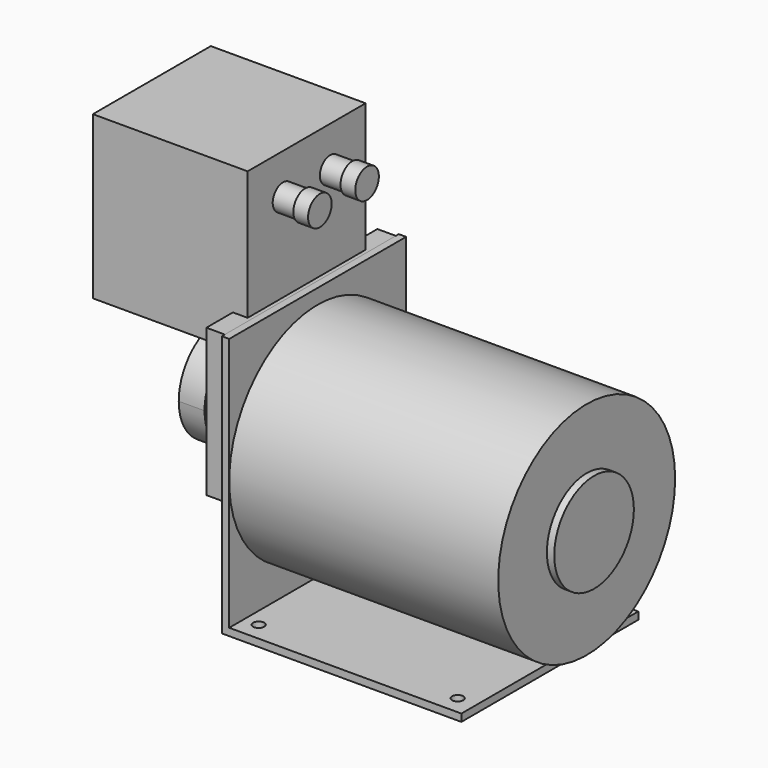
from build123d import *

# Parameters (mm, degrees)
F0_W      = 65
F0_H      = 60
F1_DEPTH  = 2
F2_W      = 2
F2_H      = 60
F3_DEPTH  = 69
F5_DEPTH  = 73
F6_R      = 13.5
F7_DEPTH  = 2
F8_W      = 58
F8_H      = 40
F9_DEPTH  = 5
F10_W     = 38
F10_H     = 27
F11_DEPTH = 5
F12_W     = 40
F12_H     = 44
F13_DEPTH = 38
F14_W     = 40
F14_H     = 35
F15_DEPTH = 4
F16_R     = 3.5
F17_DEPTH = 6
F18_R     = 4
F19_DEPTH = 4
F22_DEPTH = 3.5
F23_R     = 5
F24_DEPTH = 2
F25_R     = 12.5
F26_DEPTH = 12
F28_R     = 4
F29_DEPTH = 5
F30_R     = 1.5
F31_DEPTH = 25


with BuildPart() as f1:
    # F0 (on Top) → F1 (new body)
    with BuildSketch(Plane.XY):
        Rectangle(F0_W, F0_H)
    extrude(amount=F1_DEPTH)

    # F2 (on face) → F3 (join)
    with BuildSketch(Plane.XY.offset(2)):
        with Locations((-31.5, 0)):
            Rectangle(F2_W, F2_H)
    extrude(amount=F3_DEPTH)

    # F30 (on face) → F31 (cut)
    with BuildSketch(Plane(origin=(0, 0, 0), x_dir=(1, 0, 0), z_dir=(0, 0, -1))):
        with Locations((27.5, 25)):
            Circle(F30_R)
        with Locations((27.5, -25)):
            Circle(F30_R)
        with Locations((-26.5, 25)):
            Circle(F30_R)
        with Locations((-26.5, -25)):
            Circle(F30_R)
    extrude(amount=-F31_DEPTH, mode=Mode.SUBTRACT)


with BuildPart() as f5:
    # F4 (on face) → F5 (new body)
    with BuildSketch(Plane.YZ.offset(-30.5)):
        with BuildLine():
            ThreePointArc((-30, 37), (0, 7), (30, 37))
            ThreePointArc((30, 37), (0, 67), (-30, 37))
        make_face()
    extrude(amount=F5_DEPTH)

    # F6 (on face) → F7 (join)
    with BuildSketch(Plane.YZ.offset(42.5)):
        with Locations((0, 37)):
            Circle(F6_R)
    extrude(amount=F7_DEPTH)


with BuildPart() as f9:
    # F8 (on face) → F9 (new body)
    with BuildSketch(Plane(origin=(-32.5, 0, 0), x_dir=(0, -1, 0), z_dir=(-1, 0, 0))):
        with Locations((0, 51)):
            Rectangle(F8_W, F8_H)
    extrude(amount=F9_DEPTH)

    # F10 (on face) → F11 (cut, through all)
    with BuildSketch(Plane(origin=(-37.5, 0, 0), x_dir=(0, -1, 0), z_dir=(-1, 0, 0))):
        with Locations((0, 44.5)):
            Rectangle(F10_W, F10_H)
    extrude(amount=-F11_DEPTH, mode=Mode.SUBTRACT)

    # F12 (on face) → F13 (join)
    with BuildSketch(Plane(origin=(-37.5, 0, 0), x_dir=(0, -1, 0), z_dir=(-1, 0, 0))):
        with Locations((0, 84)):
            Rectangle(F12_W, F12_H)
    extrude(amount=F13_DEPTH)

    # F14 (on face) → F15 (join)
    with BuildSketch(Plane.YZ.offset(-37.5)):
        with Locations((0, 88.5)):
            Rectangle(F14_W, F14_H)
    extrude(amount=F15_DEPTH)

    # F16 (on face) → F17 (join)
    with BuildSketch(Plane.YZ.offset(-33.5)):
        with Locations((8, 95)):
            Circle(F16_R)
        with Locations((-8, 95)):
            Circle(F16_R)
    extrude(amount=F17_DEPTH)

    # F18 (on face) → F19 (join)
    with BuildSketch(Plane.YZ.offset(-27.5)):
        with Locations((8, 95)):
            Circle(F18_R)
        with Locations((-8, 95)):
            Circle(F18_R)
    extrude(amount=F19_DEPTH)


with BuildPart() as f22:
    # F21 (on offset) → F22 (new body, symmetric)
    with BuildSketch(Plane(origin=(-53.5, 0, 0), x_dir=(0, -1, 0), z_dir=(-1, 0, 0))):
        with BuildLine():
            Line((4, 43.0200397968), (4, 54.416407865))
            ThreePointArc((4, 54.416407865), (0, 55), (-4, 54.416407865))
            Line((-4, 54.416407865), (-4, 43.0200397968))
            Line((-4, 43.0200397968), (4, 43.0200397968))
        make_face()
        with BuildLine():
            ThreePointArc((-4, 54.416407865), (-8.3666002653, 29.7750278397), (14, 41))
            ThreePointArc((14, 41), (11.2249721603, 49.3666002653), (4, 54.416407865))
            Line((4, 54.416407865), (4, 43.0200397968))
            Line((4, 43.0200397968), (-4, 43.0200397968))
            Line((-4, 43.0200397968), (-4, 54.416407865))
        make_face()
        with BuildLine():
            ThreePointArc((-4, 54.416407865), (0, 55), (4, 54.416407865))
            Line((4, 54.416407865), (4, 65.0006011128))
            Line((4, 65.0006011128), (-4, 65.0006011128))
            Line((-4, 65.0006011128), (-4, 54.416407865))
        make_face()
    extrude(amount=F22_DEPTH, both=True)

    # F23 (on face) → F24 (join)
    with BuildSketch(Plane.YZ.offset(-50)):
        with Locations((0, 41)):
            Circle(F23_R)
    extrude(amount=F24_DEPTH)

    # F25 (on face) → F26 (join)
    with BuildSketch(Plane.YZ.offset(-48)):
        with Locations((0, 34.8997488618)):
            Circle(F25_R)
    extrude(amount=F26_DEPTH)


with BuildPart() as f29:
    # F28 (on offset) → F29 (new body)
    with BuildSketch(Plane.XZ.offset(-32)):
        with Locations((34.3298651278, 37)):
            Circle(F28_R)
    extrude(amount=F29_DEPTH)


solid = Compound([f1.part, f5.part, f9.part, f22.part, f29.part])
